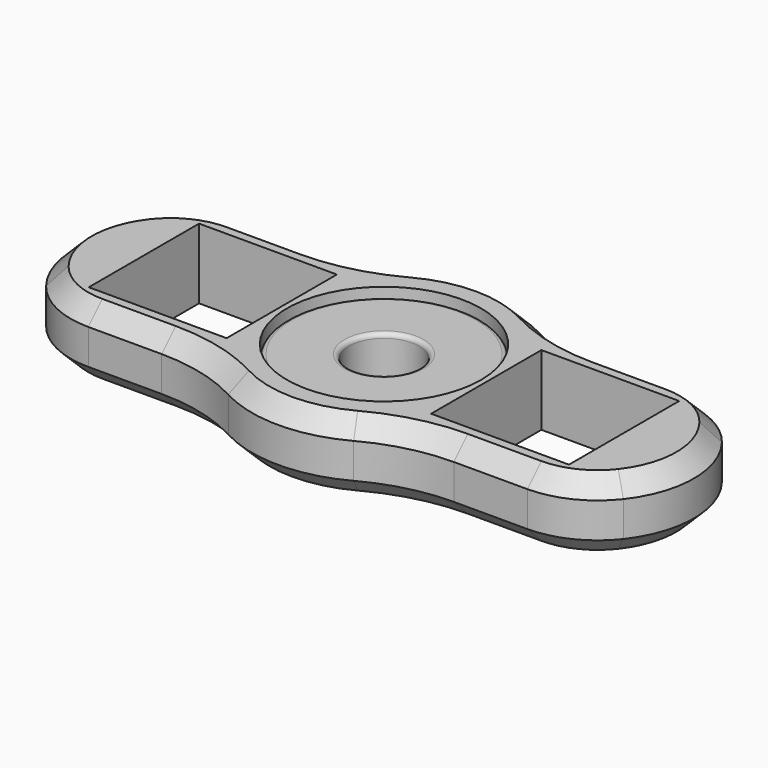
from build123d import *

# Parameters (mm, degrees)
F0_R     = 11
F0_R_2   = 4
F1_DEPTH = 7
F3_R     = 0.5
F2_R     = 11.05
F4_DEPTH = 8
F5_R     = 20
F6_R     = 10
F7_SIZE  = 2


# Not quite as in the source:
# - a feature names something its author has since deleted; it is built from what else it names


with BuildPart() as f1:
    # F0 (on Top) → F1 (new body)
    with BuildSketch(Plane.XY):
        Circle(F0_R)
        Circle(F0_R_2, mode=Mode.SUBTRACT)
    extrude(amount=F1_DEPTH)

    # F3
    f3_edges = [f1.edges().sort_by_distance(p)[0] for p in [
        (-11, 0, 0),
        (-4, 0, 0),
        (-11, 0, 7),
        (-4, 0, 7),
    ]]
    fillet(f3_edges, radius=F3_R)


with BuildPart() as f4:
    # F2 (on face) → F4 (new body)
    with BuildSketch(Plane(origin=(0, 0, 0), x_dir=(1, 0, 0), z_dir=(0, 0, -1))):
        with BuildLine():
            ThreePointArc((12.8405607354, 7.85), (11.731454134, 9.4273794822), (10.429765098, 10.85))
            ThreePointArc((10.429765098, 10.85), (0, 15.05), (-10.429765098, 10.85))
            ThreePointArc((-10.429765098, 10.85), (-11.731454134, 9.4273794822), (-12.8405607354, 7.85))
            Line((-12.8405607354, 7.85), (-11.65, 7.85))
            Line((-11.65, 7.85), (-11.65, -7.85))
            Line((-11.65, -7.85), (-12.8405607354, -7.85))
            ThreePointArc((-12.8405607354, -7.85), (-11.731454134, -9.4273794822), (-10.429765098, -10.85))
            ThreePointArc((-10.429765098, -10.85), (0, -15.05), (10.429765098, -10.85))
            ThreePointArc((10.429765098, -10.85), (11.731454134, -9.4273794822), (12.8405607354, -7.85))
            Line((12.8405607354, -7.85), (11.65, -7.85))
            Line((11.65, -7.85), (11.65, 7.85))
            Line((11.65, 7.85), (12.8405607354, 7.85))
        make_face()
        Circle(F2_R, mode=Mode.SUBTRACT)
        with BuildLine():
            Line((23, 10.85), (10.429765098, 10.85))
            ThreePointArc((10.429765098, 10.85), (11.731454134, 9.4273794822), (12.8405607354, 7.85))
            Line((12.8405607354, 7.85), (27.35, 7.85))
            Line((27.35, 7.85), (27.35, -7.85))
            Line((27.35, -7.85), (12.8405607354, -7.85))
            ThreePointArc((12.8405607354, -7.85), (11.731454134, -9.4273794822), (10.429765098, -10.85))
            Line((10.429765098, -10.85), (23, -10.85))
            Line((23, -10.85), (27.35, -10.85))
            ThreePointArc((27.35, -10.85), (35.3, 0), (27.35, 10.85))
            Line((27.35, 10.85), (23, 10.85))
        make_face()
        with BuildLine():
            ThreePointArc((-12.8405607354, 7.85), (-11.731454134, 9.4273794822), (-10.429765098, 10.85))
            Line((-10.429765098, 10.85), (-23, 10.85))
            Line((-23, 10.85), (-27.35, 10.85))
            ThreePointArc((-27.35, 10.85), (-35.3, 0), (-27.35, -10.85))
            Line((-27.35, -10.85), (-23, -10.85))
            Line((-23, -10.85), (-10.429765098, -10.85))
            ThreePointArc((-10.429765098, -10.85), (-11.731454134, -9.4273794822), (-12.8405607354, -7.85))
            Line((-12.8405607354, -7.85), (-27.35, -7.85))
            Line((-27.35, -7.85), (-27.35, 7.85))
            Line((-27.35, 7.85), (-12.8405607354, 7.85))
        make_face()
    extrude(amount=-F4_DEPTH)

    # F5
    f5_edges = [f4.edges().sort_by_distance(p)[0] for p in [
        (10.429765, -10.85, 4),
        (10.429765, 10.85, 4),
        (-10.429765, 10.85, 4),
        (-10.429765, -10.85, 4),
    ]]
    fillet(f5_edges, radius=F5_R)

    # F6
    f6_edges = [f4.edges().sort_by_distance(p)[0] for p in [
        (-27.35, -10.85, 4),
        (-27.35, 10.85, 4),
        (27.35, 10.85, 4),
        (27.35, -10.85, 4),
    ]]
    fillet(f6_edges, radius=F6_R)

    # F7
    f7_edges = [f4.edges().sort_by_distance(p)[0] for p in [
        (35.3, 0, 8),
        (-29.38625, -9.840049, 8),
        (-35.3, 0, 0),
        (35.3, 0, 0),
    ]]
    chamfer(f7_edges, length=F7_SIZE)


solid = Compound([f1.part, f4.part])
